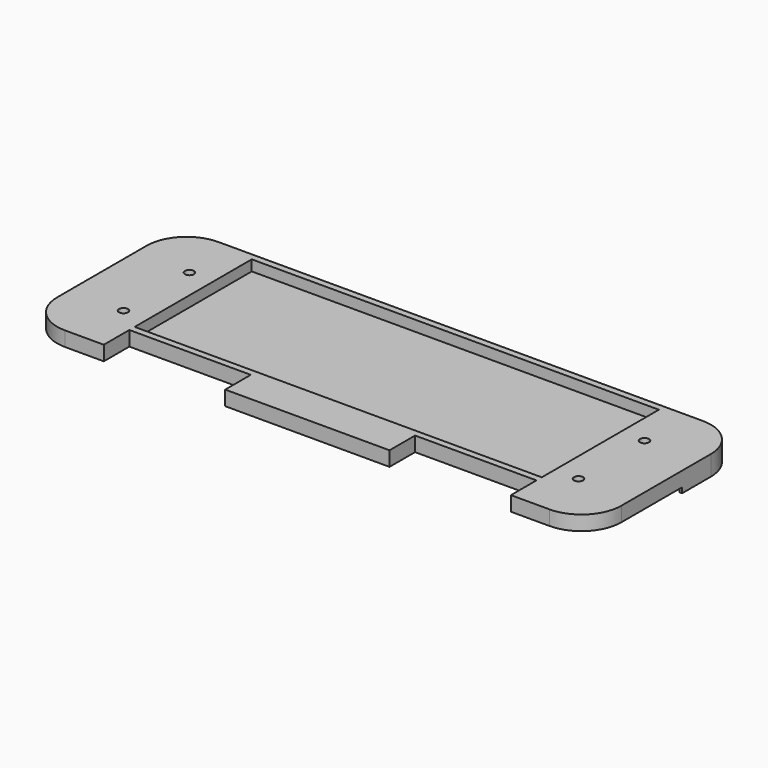
from build123d import *
from build123d import SkipClean  # not in build123d's __all__

# Parameters (mm, degrees)
F0_W      = 212
F0_H      = 72
F1_DEPTH  = 5.5
F2_R      = 15
F3_W      = 45.625
F3_H      = 5.5
F4_DEPTH  = 12
F6_DEPTH  = 2
F7_R      = 10.5
F8_R      = 11.5
F9_R      = 14
F10_R     = 15
F11_W     = 153
F11_H     = 55
F12_DEPTH = 4
F14_D     = 3.4
F15_W     = 94
F15_H     = 10.6
F16_DEPTH = 7.5
F18_DEPTH = 94


# Not quite as in the source:
# - a feature names something its author has since deleted; it is built from what else it names


with BuildPart() as f1:
    # F0 (on Top) → F1 (new body)
    with BuildSketch(Plane.XY):
        Rectangle(F0_W, F0_H)
    extrude(amount=F1_DEPTH)

    # F2
    f2_edges = [f1.edges().sort_by_distance(p)[0] for p in [
        (-106, -36, 2.75),
        (106, -36, 2.75),
    ]]
    fillet(f2_edges, radius=F2_R)

    # F3 (on face) → F4 (cut)
    with BuildSketch(Plane.XZ.offset(36)):
        with Locations((-53.6875, 2.75)):
            Rectangle(F3_W, F3_H)
        with Locations((53.6875, 2.75)):
            Rectangle(F3_W, F3_H)
    extrude(amount=-F4_DEPTH, mode=Mode.SUBTRACT)

    # F5 (on face) → F6 (join)
    with BuildSketch(Plane(origin=(0, 0, 0), x_dir=(1, 0, 0), z_dir=(0, 0, -1))):
        Polygon((-105, -7.5), (-106, -7.5), (-106, -36), (106, -36), (106, -7.5), (105, -7.5), (105, -35), (-105, -35), align=None)
        Polygon((101.5, -31.5), (-101.5, -31.5), (-101.5, -7.5), (-102.5, -7.5), (-102.5, -32.5), (102.5, -32.5), (102.5, -7.5), (101.5, -7.5), align=None)
    extrude(amount=F6_DEPTH)

    # F7
    f7_edges = [f1.edges().sort_by_distance(p)[0] for p in [
        (101.5, 31.5, -1),
        (-101.5, 31.5, -1),
    ]]
    fillet(f7_edges, radius=F7_R)

    # F8
    f8_edges = [f1.edges().sort_by_distance(p)[0] for p in [
        (102.5, 32.5, -1),
        (-102.5, 32.5, -1),
    ]]
    fillet(f8_edges, radius=F8_R)

    # F9
    f9_edges = [f1.edges().sort_by_distance(p)[0] for p in [
        (105, 35, -1),
        (-105, 35, -1),
    ]]
    fillet(f9_edges, radius=F9_R)

    # F10
    f10_edges = [f1.edges().sort_by_distance(p)[0] for p in [
        (106, 36, 1.75),
        (-106, 36, 1.75),
    ]]
    fillet(f10_edges, radius=F10_R)

    # F11 (on face) → F12 (cut)
    with BuildSketch(Plane.XY.offset(5.5)):
        with Locations((0, 6)):
            Rectangle(F11_W, F11_H)
    extrude(amount=-F12_DEPTH, mode=Mode.SUBTRACT)

    # F14 (through all)
    with Locations(Plane.XY.offset(5.5)):
        with Locations((-85.5, 15.5), (85.5, 15.5), (85.5, -15.5), (-85.5, -15.5)):
            Hole(F14_D / 2)

    # F15 (on face) → F16 (join)
    with BuildSketch(Plane(origin=(0, 0, 0), x_dir=(1, 0, 0), z_dir=(0, 0, -1))):
        with Locations((0, 6.3955)):
            Rectangle(F15_W, F15_H)
        with Locations((0, -6.3955)):
            Rectangle(F15_W, F15_H)
    extrude(amount=F16_DEPTH)

    # F17 (on face) → F18 (cut)
    with BuildSketch(Plane.YZ.offset(47)):
        with BuildLine():
            Line((11.6955, -7.5), (11.6955, 0))
            ThreePointArc((11.6955, 0), (8.867073, -1.171573), (7.6955, -4))
            Line((7.6955, -4), (7.6955, -7.5))
            Line((7.6955, -7.5), (11.6955, -7.5))
        make_face()
        with BuildLine():
            Line((-1.095439, -7.5), (-1.095439, 0))
            ThreePointArc((-1.095439, 0), (-3.923866, -1.171573), (-5.095439, -4))
            Line((-5.095439, -4), (-5.095439, -7.5))
            Line((-5.095439, -7.5), (-1.095439, -7.5))
        make_face()
        with BuildLine():
            Line((5.0955, -7.5), (5.0955, -4))
            ThreePointArc((5.0955, -4), (3.923927, -1.171573), (1.0955, 0))
            Line((1.0955, 0), (1.0955, -7.5))
            Line((1.0955, -7.5), (5.0955, -7.5))
        make_face()
        with BuildLine():
            Line((-7.695949, -7.5), (-7.695949, -4))
            ThreePointArc((-7.695949, -4), (-8.867522, -1.171573), (-11.695949, 0))
            Line((-11.695949, 0), (-11.695949, -7.5))
            Line((-11.695949, -7.5), (-7.695949, -7.5))
        make_face()
    with SkipClean():  # cleaning this boolean's faces spoils the solid; the shape is the same uncleaned
        extrude(amount=-F18_DEPTH, mode=Mode.SUBTRACT)


solid = f1.part
